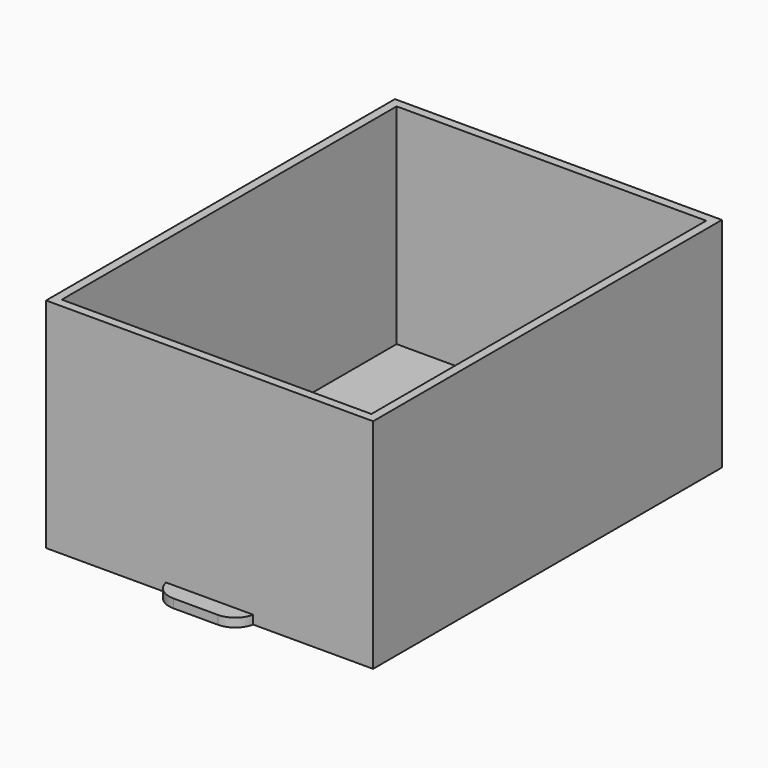
from build123d import *

# Parameters (mm, degrees)
F2_W        = 75
F2_H        = 100
F3_DEPTH    = 50
F4_T        = -2
F5_W        = 20
F5_H        = 2
F6_DEPTH    = 4
F7_T1_DEPTH = 26.4948974279


# Not quite as in the source:
# - a fillet or chamfer that OpenCascade refuses, or shapes differently, is made with other operations: its cross-section is extruded or revolved along the edge and cut away or added


with BuildPart() as f3:
    # F2 (on Top) → F3 (new body)
    with BuildSketch(Plane.XY):
        Rectangle(F2_W, F2_H)
    extrude(amount=-F3_DEPTH)

    # F4
    f4_openings = [f3.faces().sort_by_distance(p)[0] for p in [
        (0, 0, 0),
    ]]
    offset(amount=F4_T, openings=f4_openings)

    # F5 (on face) → F6 (join)
    with BuildSketch(Plane.XZ.offset(50)):
        with Locations((0, -49)):
            Rectangle(F5_W, F5_H)
    extrude(amount=F6_DEPTH)

    # F7: fillet of radius 5 on 2 edges, made by hand

    # F7_s2 → F7_t1 (cut)
    with BuildSketch(Plane.XY.offset(-62.2474487139)):
        with BuildLine():
            ThreePointArc((10, -50), (8.2632981746, -52.8729833462), (5.1010205144, -54))
            Line((5.1010205144, -54), (10, -54))
            Line((10, -54), (10, -50))
        make_face()
        with BuildLine():
            ThreePointArc((-10, -50), (-8.2632981746, -52.8729833462), (-5.1010205144, -54))
            Line((-5.1010205144, -54), (-10, -54))
            Line((-10, -54), (-10, -50))
        make_face()
    extrude(amount=F7_T1_DEPTH, mode=Mode.SUBTRACT)


solid = f3.part
